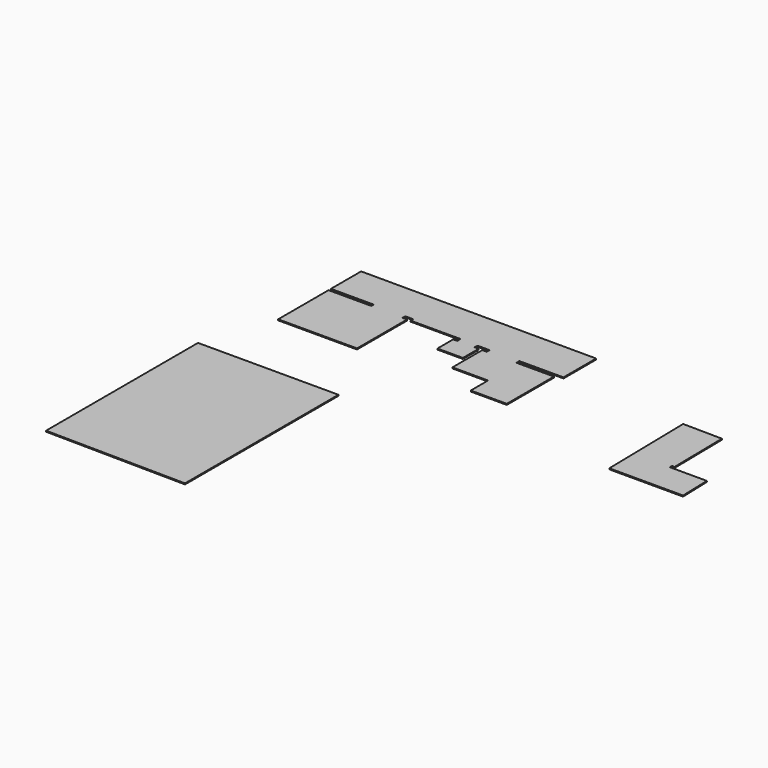
from build123d import *

# Parameters (mm, degrees)
F1_DEPTH = 25.4
F2_DEPTH = 25.4
F3_DEPTH = 25.4


with BuildPart() as f1:
    # F0 (on Top) → F1 (new body)
    with BuildSketch(Plane.XY):
        Polygon((-2728.2330813421, -222.2274847333), (-2726.1031090565, -5017.4901109881), (816.1276547891, -5062.9762998701), (816.1276547891, -222.2274847333), align=None)
    extrude(amount=F1_DEPTH)


with BuildPart() as f2:
    # F0 (on Top) → F2 (new body)
    with BuildSketch(Plane.XY):
        Polygon((7888.2079124451, 3035.3169441223), (6899.0507125854, 3048.196554184), (6945.4174041748, 662.8842353821), (8805.2396774292, 662.8842353821), (8782.0558547974, 1443.3914422989), (7844.4170951843, 1443.3914422989), (7844.4170951843, 1511.5010225121), (7911.8941330612, 1511.5010225121), align=None)
    extrude(amount=F2_DEPTH)


with BuildPart() as f3:
    # F0 (on Top) → F3 (new body)
    with BuildSketch(Plane.XY):
        Polygon((3815.2096271515, 4158.4286689758), (-2124.28855896, 4169.2004203796), (-2124.28855896, 3216.2303924561), (-1044.7806119919, 3216.2303924561), (-1044.7806119919, 3141.6304111481), (-2124.28855896, 3141.6304111481), (-2124.28855896, 1552.127122879), (-134.369879961, 1552.127122879), (-134.369879961, 3127.103805542), (-250.0150203705, 3127.103805542), (-250.0150203705, 3216.2303924561), (-47.8258170187, 3216.2303924561), (-47.8258170187, 3138.5490894318), (1206.9922685623, 3138.5490894318), (1206.9922685623, 3036.0553264618), (1105.9012413025, 3036.0553264618), (1105.9012413025, 2538.1681919098), (1749.3126392365, 2538.1681919098), (1749.3126392365, 3036.0553264618), (1646.2754011154, 3036.0553264618), (1646.2754011154, 3125.4806518555), (1952.8112411499, 3125.4806518555), (1952.8112411499, 3036.0553264618), (1839.4702672958, 3036.0553264618), (1839.4702672958, 2095.1080322266), (2738.4703159332, 2095.1080322266), (2738.4703159332, 1549.0103960037), (3647.7742195129, 1549.0103960037), (3647.7742195129, 3036.0553264618), (2702.4071216583, 3036.0553264618), (2702.4071216583, 3128.0562877655), (3815.2096271515, 3128.0562877655), align=None)
    extrude(amount=F3_DEPTH)


solid = Compound([f1.part, f2.part, f3.part])
